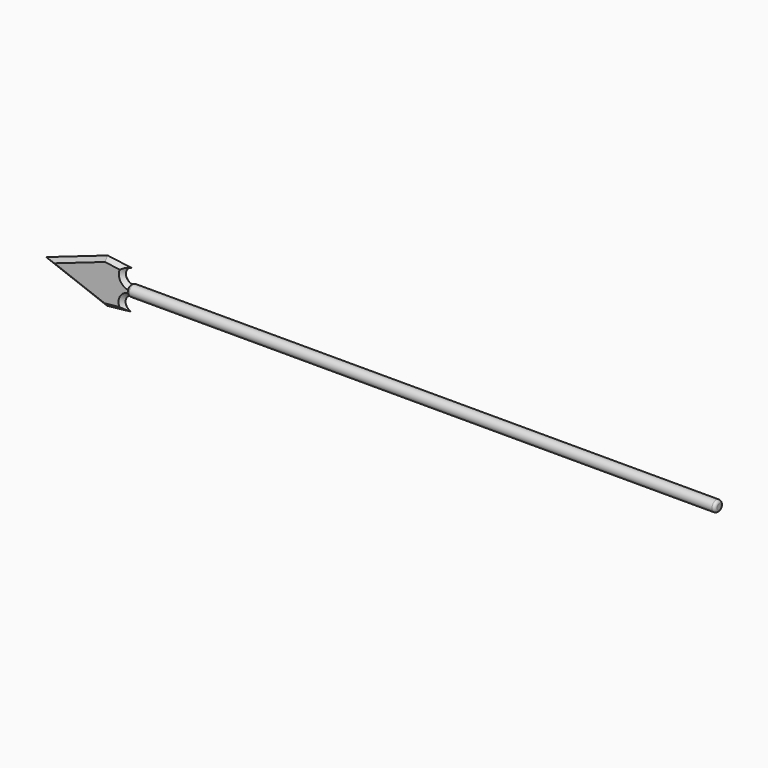
from build123d import *

# Parameters (mm, degrees)
F0_W     = 533.4084779024
F0_H     = 4.8805493861
F3_R     = 2.54
F4_DEPTH = 3.556
F5_SIZE  = 3.55599
F6_R     = 2.54


# Not quite as in the source:
# - a fillet or chamfer is up to 0.001 mm smaller than in the source, because OpenCascade refuses the exact size
# - a feature names something its author has since deleted; it is built from what else it names


with BuildPart() as f1:
    # F0 (on Front) → F1 (revolve)
    with BuildSketch(Plane.XZ):
        with Locations((119.7407469153, 11.39604114)):
            Rectangle(F0_W, F0_H)
    revolve(axis=Axis((119.7407469153, 0, 13.836315833), (1, 0, 0)))

    # F3
    f3_edges = [f1.edges().sort_by_distance(p)[0] for p in [
        (386.444986, 0, 18.716865),
    ]]
    fillet(f3_edges, radius=F3_R)

    # F6
    f6_edges = [f1.edges().sort_by_distance(p)[0] for p in [
        (-146.963492, 0, 18.716865),
    ]]
    fillet(f6_edges, radius=F6_R)


with BuildPart() as f4:
    # F2 (on Front) → F4 (new body, symmetric)
    with BuildSketch(Plane.XZ):
        with BuildLine():
            ThreePointArc((-146.3349759579, -3.7328371559), (-151.6437669731, 3.1876916726), (-145.2257782221, 9.0941628441))
            Line((-145.2257782221, 9.0941628441), (-145.2257782221, 13.7774241157))
            Line((-145.2257782221, 13.7774241157), (-145.1088434278, 18.4592253066))
            ThreePointArc((-145.1088434278, 18.4592253066), (-151.3773545538, 24.5241036708), (-145.8974222536, 31.3099214766))
            Line((-145.8974222536, 31.3099214766), (-167.8842370803, 34.2305423366))
            Line((-167.8842370803, 34.2305423366), (-223.7618170531, 14.7580471046))
            Line((-223.7618170531, 14.7580471046), (-168.3878600597, -6.1035659938))
            Line((-168.3878600597, -6.1035659938), (-146.3349759579, -3.7328371559))
        make_face()
    extrude(amount=F4_DEPTH, both=True)

    # F5 (size 3.556 in the source; OpenCascade refuses exactly that, so slightly less here)
    f5_edges = [f4.edges().sort_by_distance(p)[0] for p in [
        (-157.361418, 3.556, -4.918202),
        (-196.074839, 3.556, 4.327241),
        (-157.361418, -3.556, -4.918202),
        (-196.074839, -3.556, 4.327241),
        (-151.643767, -3.556, 3.187692),
        (-151.643767, 3.556, 3.187692),
        (-151.377355, -3.556, 24.524104),
        (-156.89083, -3.556, 32.770232),
        (-195.823027, -3.556, 24.494295),
        (-151.377355, 3.556, 24.524104),
        (-195.823027, 3.556, 24.494295),
        (-156.89083, 3.556, 32.770232),
    ]]
    chamfer(f5_edges, length=F5_SIZE)


solid = Compound([f1.part, f4.part])
